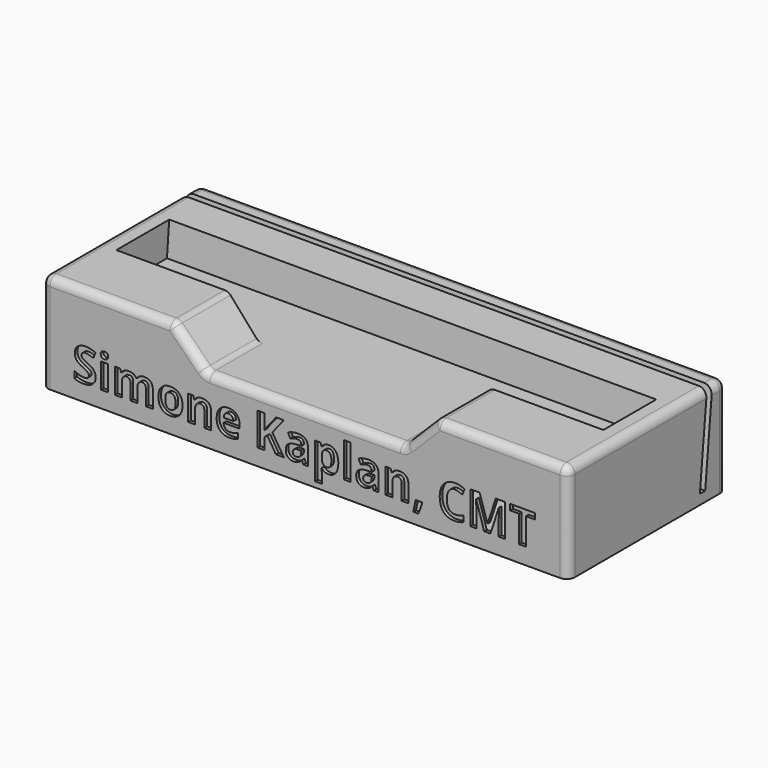
from build123d import *

# Parameters (mm, degrees)
F0_W         = 30
F0_H         = 15
F1_DEPTH     = 80
F3_DEPTH     = 80
F5_REACH     = 70.3122887415
F7_DEPTH     = 3
F8_START     = -77
F8_DEPTH     = 3
F9_TEXT_SIZE = 6.9444444444
F10_DEPTH    = 0.5
F11_R        = 1.25


# Not quite as in the source:
# - Text() gives the source's letters only with a copy of the font that has no kerning and outlines rounded to 1/6400 em; it was checked with that copy


with BuildPart() as f1:
    # F0 (on Right) → F1 (new body)
    with BuildSketch(Plane.YZ):
        with Locations((15, 7.5)):
            Rectangle(F0_W, F0_H)
    extrude(amount=F1_DEPTH)

    # F2 (on face) → F3 (cut)
    with BuildSketch(Plane.YZ.offset(80)):
        Polygon((20.4565425053, 15), (10.4183441299, 15), (9.9809008123, 10), (20.0190991877, 10), align=None)
        Polygon((26.9809156656, 21.2844415417), (26.3516864466, 15), (27.3566864466, 15), (27.9859156656, 21.2844415417), align=None)
        Polygon((27.3566864466, 15), (26.3516864466, 15), (25, 1.5), (26.005, 1.5), align=None)
    extrude(amount=-F3_DEPTH, mode=Mode.SUBTRACT)

    f5_end = f1.faces().sort_by_distance((40, 20.2378208465, 12.5))[0]
    # F4 (on face) → F5 (cut, up to a face of the model that its end follows)
    with BuildSketch(Plane.XZ):
        Polygon((60, 15), (20, 15), (25, 10), (55, 10), align=None)
    f5_long = extrude(amount=-F5_REACH, mode=Mode.PRIVATE)
    add(split(f5_long, bisect_by=f5_end, keep=Keep.TOP, mode=Mode.PRIVATE), mode=Mode.SUBTRACT)

    # F6 (on face) → F7 (join)
    with BuildSketch(Plane.YZ.offset(80)):
        Polygon((20.0190991877, 10), (20.4565425053, 15), (10.4183441299, 15), (9.9809008123, 10), align=None)
    extrude(amount=-F7_DEPTH)

    # F6 (on face) → F8 (join)
    with BuildSketch(Plane.YZ.offset(80).offset(F8_START)):
        Polygon((20.0190991877, 10), (20.4565425053, 15), (10.4183441299, 15), (9.9809008123, 10), align=None)
    extrude(amount=-F8_DEPTH)

    # F9 (on face) → F10 (cut)
    with BuildSketch(Plane.XZ):
        with Locations((4.6321614583, 2.5)):
            Text('Simone Kaplan, CMT', F9_TEXT_SIZE, font='Open Sans', font_style=FontStyle.BOLD, text_align=(TextAlign.LEFT, TextAlign.BOTTOM))
    extrude(amount=-F10_DEPTH, mode=Mode.SUBTRACT)

    # F11
    f11_edges = [f1.edges().sort_by_distance(p)[0] for p in [
        (10, 0, 15),
        (0, 13.175843, 15),
        (0, 0, 7.5),
        (80, 0, 7.5),
        (80, 30, 7.5),
        (20, 5.209172, 15),
        (22.5, 0, 12.5),
        (70, 0, 15),
        (80, 13.175843, 15),
        (80, 28.678343, 15),
        (0, 28.678343, 15),
        (0, 30, 7.5),
        (40, 30, 15),
        (57.5, 0, 12.5),
        (40, 0, 10),
        (25, 4.99045, 10),
        (55, 4.99045, 10),
        (60, 5.209172, 15),
    ]]
    fillet(f11_edges, radius=F11_R)


solid = f1.part
